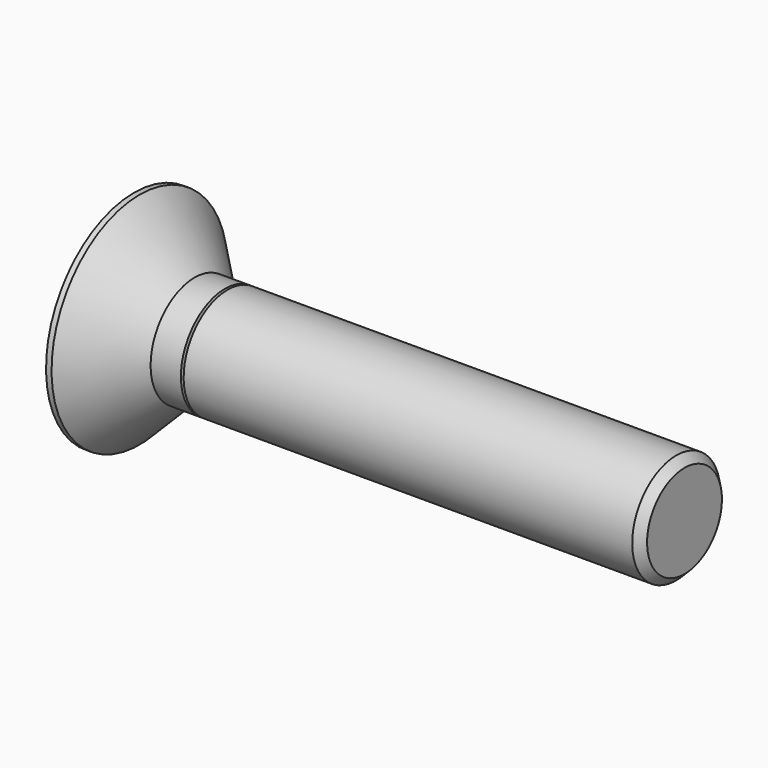
from build123d import *

# Parameters (mm, degrees)
F3_DEPTH = 4
F4_SIZE  = 4.99999


# Not quite as in the source:
# - a fillet or chamfer is up to 0.001 mm smaller than in the source, because OpenCascade refuses the exact size


with BuildPart() as f1:
    # F0 (on Front) → F1 (revolve)
    with BuildSketch(Plane.XZ):
        Polygon((5.5, 5), (5.5, 10), (0, 10), (0, 0), (50, 0), (50, 4.25), (49.25, 5), (8.5, 5), (8.375, 4.25), (8.25, 5), align=None)
    revolve(axis=Axis((25, 0, 0), (1, 0, 0)))

    # F2 (on face) → F3 (cut)
    with BuildSketch(Plane(origin=(0, 0, 0), x_dir=(0, -1, 0), z_dir=(-1, 0, 0))):
        Polygon((0, -2.8867513459), (2.5, -1.443375673), (2.5, 1.443375673), (0, 2.8867513459), (-2.5, 1.443375673), (-2.5, -1.443375673), align=None)
    extrude(amount=-F3_DEPTH, mode=Mode.SUBTRACT)

    # F4 (size 5 in the source; OpenCascade refuses exactly that, so slightly less here)
    f4_edges = [f1.edges().sort_by_distance(p)[0] for p in [
        (5.5, 0, -10),
    ]]
    chamfer(f4_edges, length=F4_SIZE)


solid = f1.part
